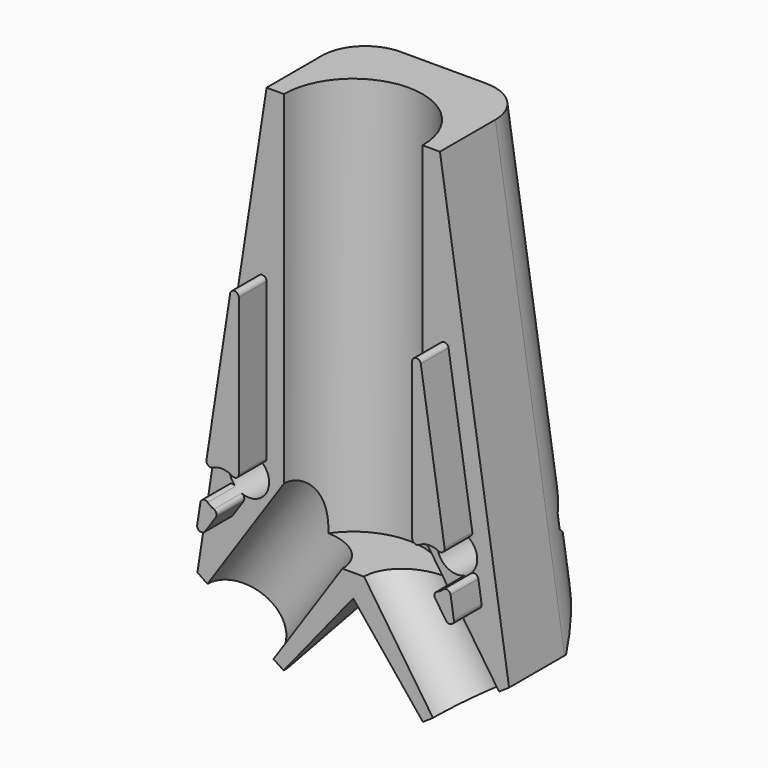
from build123d import *

# Parameters (mm, degrees)
F0_R          = 2.3
F1_DEPTH      = 13
F3_DEPTH      = 46
F6_DEPTH      = 52.2
F8_DEPTH      = 25
F10_DEPTH     = 25
F11_T1_DEPTH  = 69.4664340584
F11_T3_DEPTH  = 69.4664340584
F11_T8_DEPTH  = 31.9524083705
F11_T13_DEPTH = 31.9524083705
F11_T19_DEPTH = 31.9524083705
F11_T23_DEPTH = 31.9524083705
F15_DEPTH     = 4
F16_DEPTH     = 4
F19_DEPTH     = 28
F20_R         = 2.3
F21_DEPTH     = 25
F22_R         = 2.3
F23_DEPTH     = 25
F24_R         = 0.5


# Not quite as in the source:
# - a fillet or chamfer that OpenCascade refuses, or shapes differently, is made with other operations: its cross-section is extruded or revolved along the edge and cut away or added
# - a feature names something its author has since deleted; it is built from what else it names


with BuildPart() as f1:
    # F0 (on Front) → F1 (new body)
    with BuildSketch(Plane.XZ):
        Polygon((10, 40), (-10, 40), (-17.9806351662, -11.8325809017), (-8.0368565166, -18.5498173996), (0, -8.6111112242), (8.0368565166, -18.5498173996), (17.9806351662, -11.8325809017), align=None)
        with Locations((-12, 0)):
            Circle(F0_R, mode=Mode.SUBTRACT)
        with Locations((12, 0)):
            Circle(F0_R, mode=Mode.SUBTRACT)
    extrude(amount=-F1_DEPTH)

    # F2 (on face) → F3 (cut)
    with BuildSketch(Plane.XY.offset(40)):
        with BuildLine():
            Line((-8, 0), (8, 0))
            ThreePointArc((8, 0), (0, 8), (-8, 0))
        make_face()
    extrude(amount=-F3_DEPTH, mode=Mode.SUBTRACT)

    # F5 (on offset) → F6 (cut)
    with BuildSketch(Plane.YZ.offset(25)):
        Polygon((13, -3.9485500787), (4.1381944902, -18.5498173996), (13, -18.5498173996), align=None)
    extrude(amount=-F6_DEPTH, mode=Mode.SUBTRACT)

    # F7 (on face) → F8 (cut)
    with BuildSketch(Plane(origin=(-11.122658813, 0, -16.4652915326), x_dir=(0.8286482208, 0, -0.5597697082), z_dir=(-0.5597697082, 0, -0.8286482208))):
        with BuildLine():
            ThreePointArc((-6.8761009811, 0), (-2.2761009811, -4.6), (2.3238990189, 0))
            Line((2.3238990189, 0), (-6.8761009811, 0))
        make_face()
    extrude(amount=-F8_DEPTH, mode=Mode.SUBTRACT)

    # F9 (on face) → F10 (cut)
    with BuildSketch(Plane(origin=(11.122658813, 0, -16.4652915326), x_dir=(0.8286482208, 0, 0.5597697082), z_dir=(0.5597697082, 0, -0.8286482208))):
        with BuildLine():
            ThreePointArc((-2.3238990189, 0), (2.2761009811, -4.6), (6.8761009811, 0))
            Line((6.8761009811, 0), (-2.3238990189, 0))
        make_face()
    extrude(amount=-F10_DEPTH, mode=Mode.SUBTRACT)

    # F11: fillet of radius 5 on 4 edges, made by hand

    # F11_s2 → F11_t1 (cut)
    with BuildSketch(Plane(origin=(7.6867833124, 0, 49.9240736631), x_dir=(0, 1, 0), z_dir=(-0.152176248, 0, -0.9883533728))):
        with BuildLine():
            ThreePointArc((13, -10.9705836466), (11.5355339059, -14.5061175525), (8, -15.9705836466))
            Line((8, -15.9705836466), (13, -15.9705836466))
            Line((13, -15.9705836466), (13, -10.9705836466))
        make_face()
    extrude(amount=F11_T1_DEPTH, mode=Mode.SUBTRACT)

    # F11_s4 → F11_t3 (cut)
    with BuildSketch(Plane(origin=(2.8843579817, 0, -18.733310736), x_dir=(0, 1, 0), z_dir=(-0.152176248, 0, 0.9883533728))):
        with BuildLine():
            ThreePointArc((8, -15.9705836466), (11.5355339059, -14.5061175525), (13, -10.9705836466))
            Line((13, -10.9705836466), (13, -15.9705836466))
            Line((13, -15.9705836466), (8, -15.9705836466))
        make_face()
    extrude(amount=F11_T3_DEPTH, mode=Mode.SUBTRACT)


with BuildPart() as f11_tool6:
    # F11_s7 → F11_t8 (new body)
    with BuildSketch(Plane(origin=(4.0911710208, 3.0705977915, 5.0593097692), x_dir=(0.6002776597, -0.7997916799, 0), z_dir=(-0.5686414, -0.4267895471, -0.7032052622))):
        with BuildLine():
            ThreePointArc((-10.7347001393, -7.9787789452), (-7.9821654916, -9.2854915519), (-4.9822833283, -8.7519638303))
            Line((-4.9822833283, -8.7519638303), (-8.1340389445, -10.4154145762))
            Line((-8.1340389445, -10.4154145762), (-10.7347001393, -7.9787789452))
        make_face()
    extrude(amount=F11_T8_DEPTH)

    split(bisect_by=Plane(origin=(-4.2102294585, 0, -3.404568911), x_dir=(0, 1, 0), z_dir=(-0.7775800359, 0, -0.6287839754)), keep=Keep.TOP)


with BuildPart() as f1_1:
    add(f1.part)

    # F11_t5: cut F11_tool6
    add(f11_tool6.part, mode=Mode.SUBTRACT)


with BuildPart() as f11_tool11:
    # F11_s12 → F11_t13 (new body)
    with BuildSketch(Plane(origin=(14.0782912081, -10.566356105, -17.4097919354), x_dir=(-0.6002776597, -0.7997916799, 0), z_dir=(-0.5686414, 0.4267895471, 0.7032052622))):
        with BuildLine():
            ThreePointArc((-10.7347001393, -7.9787789452), (-7.9821654916, -9.2854915519), (-4.9822833283, -8.7519638303))
            Line((-4.9822833283, -8.7519638303), (-8.1340389445, -10.4154145762))
            Line((-8.1340389445, -10.4154145762), (-10.7347001393, -7.9787789452))
        make_face()
    extrude(amount=F11_T13_DEPTH)

    split(bisect_by=Plane(origin=(4.2102294585, 0, -3.404568911), x_dir=(0, 1, 0), z_dir=(0.7775800359, 0, -0.6287839754)), keep=Keep.TOP)


with BuildPart() as f1_2:
    add(f1_1.part)

    # F11_t10: cut F11_tool11
    add(f11_tool11.part, mode=Mode.SUBTRACT)


with BuildPart() as f11_tool17:
    # F11_s18 → F11_t19 (new body)
    with BuildSketch(Plane(origin=(14.0782912081, -10.566356105, -17.4097919354), x_dir=(-0.6002776597, -0.7997916799, 0), z_dir=(-0.5686414, 0.4267895471, 0.7032052622))):
        with BuildLine():
            ThreePointArc((-10.7347001393, -7.9787789452), (-7.9821654916, -9.2854915519), (-4.9822833283, -8.7519638303))
            Line((-4.9822833283, -8.7519638303), (-8.1340389445, -10.4154145762))
            Line((-8.1340389445, -10.4154145762), (-10.7347001393, -7.9787789452))
        make_face()
    extrude(amount=F11_T19_DEPTH)

    split(bisect_by=Plane(origin=(4.2102294585, 0, -3.404568911), x_dir=(0, 1, 0), z_dir=(-0.7775800359, 0, 0.6287839754)), keep=Keep.TOP)


with BuildPart() as f11_tool21:
    # F11_s22 → F11_t23 (new body)
    with BuildSketch(Plane(origin=(4.0911710208, 3.0705977915, 5.0593097692), x_dir=(0.6002776597, -0.7997916799, 0), z_dir=(-0.5686414, -0.4267895471, -0.7032052622))):
        with BuildLine():
            ThreePointArc((-10.7347001393, -7.9787789452), (-7.9821654916, -9.2854915519), (-4.9822833283, -8.7519638303))
            Line((-4.9822833283, -8.7519638303), (-8.1340389445, -10.4154145762))
            Line((-8.1340389445, -10.4154145762), (-10.7347001393, -7.9787789452))
        make_face()
    extrude(amount=F11_T23_DEPTH)

    split(bisect_by=Plane(origin=(-4.2102294585, 0, -3.404568911), x_dir=(0, 1, 0), z_dir=(0.7775800359, 0, 0.6287839754)), keep=Keep.TOP)


with BuildPart() as f11_tool17_1:
    add(f11_tool17.part)

    # F11_t25: intersect F11_tool21
    add(f11_tool21.part, mode=Mode.INTERSECT)


with BuildPart() as f1_3:
    add(f1_2.part)

    # F11_t15: cut F11_tool17
    add(f11_tool17_1.part, mode=Mode.SUBTRACT)

    # F14 (on face) → F15 (join)
    with BuildSketch(Plane.XZ):
        Polygon((-15.1459260242, -6.5643846345), (-10, 1.0533238305), (-10, 26.8573445146), align=None)
    extrude(amount=F15_DEPTH)

    # F12 (on face) → F16 (join)
    with BuildSketch(Plane.XZ):
        Polygon((15.1459253956, -6.5643830302), (10.0000003771, 26.8573395869), (10.0000003771, 1.0533239459), align=None)
    extrude(amount=F16_DEPTH)

    # F18 (on offset) → F19 (cut)
    with BuildSketch(Plane(origin=(0, 38, 0), x_dir=(-1, 0, 0), z_dir=(0, 1, 0))):
        Polygon((-9.9215390309, 3.6), (-14.0784609691, 3.6), (-16.1569219382, 0), (-14.0784609691, -3.6), (-9.9215390309, -3.6), (-7.8430780618, 0), align=None)
        Polygon((14.0784609691, 3.6), (9.9215390309, 3.6), (7.8430780618, 0), (9.9215390309, -3.6), (14.0784609691, -3.6), (16.1569219382, 0), align=None)
    extrude(amount=-F19_DEPTH, mode=Mode.SUBTRACT)

    # F20 (on face) → F21 (cut)
    with BuildSketch(Plane.XZ.offset(4)):
        with Locations((12, 0)):
            Circle(F20_R)
    extrude(amount=-F21_DEPTH, mode=Mode.SUBTRACT)

    # F22 (on face) → F23 (cut)
    with BuildSketch(Plane.XZ.offset(4)):
        with Locations((-12, 0)):
            Circle(F22_R)
    extrude(amount=-F23_DEPTH, mode=Mode.SUBTRACT)

    # F24
    f24_edges = [f1_3.edges().sort_by_distance(p)[0] for p in [
        (-10, -2, 26.857345),
        (10, -2, 26.85734),
        (-15.145926, -2, -6.564385),
        (15.145925, -2, -6.564383),
        (-10, -2, 1.135782),
        (-13.946588, -2, 1.22507),
        (-14.224942, -2, -0.582781),
        (10, -2, 1.135782),
        (13.946587, -2, 1.22507),
        (14.224941, -2, -0.582782),
        (12.255618, -2, -2.285751),
        (-12.255617, -2, -2.285751),
    ]]
    fillet(f24_edges, radius=F24_R)


solid = f1_3.part
